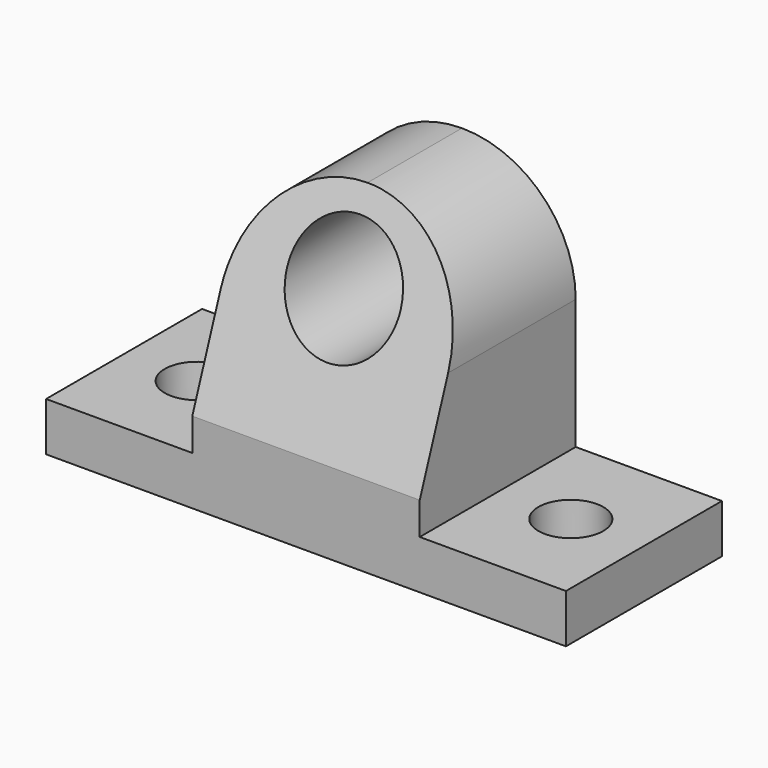
from build123d import *

# Parameters (mm, degrees)
F0_W        = 22.5
F0_H        = 15
F0_R        = 17.5
F1_DEPTH    = 60
F2_R        = 10
F3_DEPTH    = 75.9
F4_T1_DEPTH = 407.2453152316
F5_R        = 34.99999


# Not quite as in the source:
# - a fillet or chamfer that OpenCascade refuses, or shapes differently, is made with other operations: its cross-section is extruded or revolved along the edge and cut away or added
# - a fillet or chamfer is up to 0.001 mm smaller than in the source, because OpenCascade refuses the exact size


with BuildPart() as f1:
    # F0 (on Front) → F1 (new body)
    with BuildSketch(Plane.XZ):
        Polygon((-24.4408938289, -40.7930500805), (10.5591061711, -40.7930500805), (13.0723165348, -40.7930500805), (45.5591061711, -40.7930500805), (45.5591061711, -35.7930500805), (-24.4408938289, -35.7930500805), align=None)
        Polygon((13.0723165348, -40.7930500805), (10.5591061711, -40.7930500805), (-24.4408938289, -40.7930500805), (-46.9408938289, -40.7930500805), (-46.9408938289, -55.7930500805), (68.0591061711, -55.7930500805), (68.0591061711, -40.7930500805), (45.5591061711, -40.7930500805), align=None)
        with Locations((-58.1908938289, -48.2930500805)):
            Rectangle(F0_W, F0_H)
        Polygon((-24.4408938289, 9.2069499195), (-24.4408938289, -35.7930500805), (45.5591061711, -35.7930500805), (45.5591061711, 9.2069499195), (45.5591061711, 34.2069499195), (-24.4408938289, 34.2069499195), align=None)
        with Locations((10.5591061711, 9.2069499195)):
            Circle(F0_R, mode=Mode.SUBTRACT)
        with Locations((79.3091061711, -48.2930500805)):
            Rectangle(F0_W, F0_H)
    extrude(amount=F1_DEPTH)

    # F2 (on Top) → F3 (cut)
    with BuildSketch(Plane.XY):
        with Locations((-46.9408938289, -30)):
            Circle(F2_R)
        with Locations((68.0591061711, -30)):
            Circle(F2_R)
    extrude(amount=-F3_DEPTH, mode=Mode.SUBTRACT)

    # F4: chamfer of 65 x 23.6580652273 on 1 edges, made by hand

    # F4_s2 → F4_t1 (cut)
    with BuildSketch(Plane.YZ.offset(-193.0635514447)):
        Polygon((-60, -30.7930500805), (-36.3419347727, 34.2069499195), (-60, 34.2069499195), align=None)
    extrude(amount=F4_T1_DEPTH, mode=Mode.SUBTRACT)

    # F5 (radius 35 in the source; OpenCascade refuses exactly that, so slightly less here)
    f5_edges = [f1.edges().sort_by_distance(p)[0] for p in [
        (45.559106, -18.170967, 34.20695),
        (-24.440894, -18.170967, 34.20695),
    ]]
    fillet(f5_edges, radius=F5_R)


solid = f1.part
